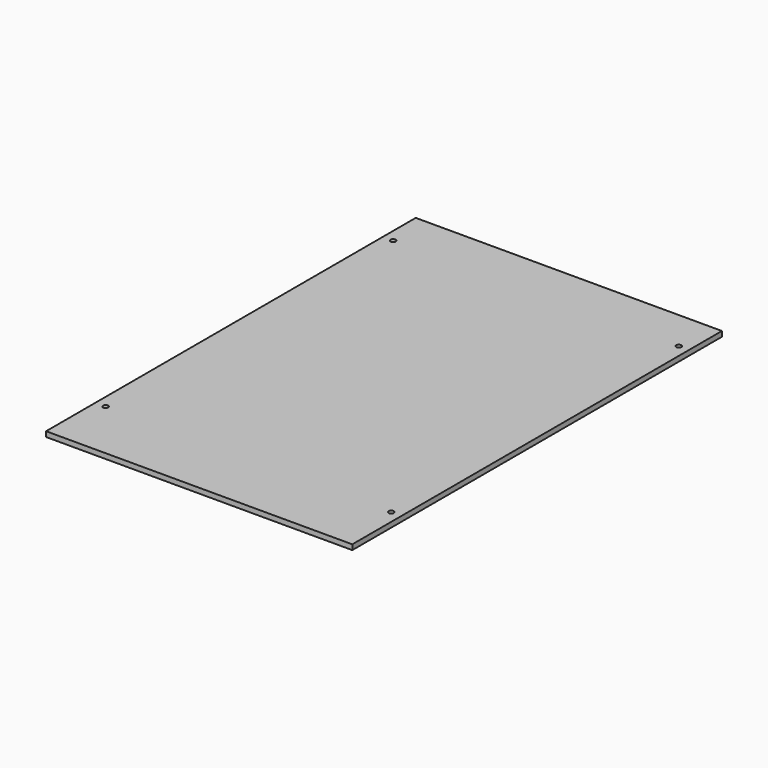
from build123d import *

# Parameters (mm, degrees)
F0_W     = 378.7394
F0_H     = 571.5
F1_DEPTH = 6.35
F3_DEPTH = 6.351


# Not quite as in the source:
# - a length typed as a fraction of an inch, garbled in the dataset ("3 / 203.2 mm" for 3/8 in), is restored


with BuildPart() as f1:
    # F0 (on Top) → F1 (new body)
    with BuildSketch(Plane.XY):
        with Locations((-22.0819663584, 200.0282000497)):
            Rectangle(F0_W, F0_H)
    extrude(amount=F1_DEPTH)

    # F2 (on face) → F3 (cut, through all)
    with BuildSketch(Plane.XY.offset(6.35)):
        with BuildLine():
            ThreePointArc((-201.9266663584, 434.9782000497), (-198.7516663584, 431.8032000497), (-195.5766663584, 434.9782000497))
            ThreePointArc((-195.5766663584, 434.9782000497), (-195.6025010735, 435.3824066906), (-195.679584789, 435.7800353388))
            Line((-195.679584789, 435.7800353388), (-198.7516663584, 434.9782000497))
            Line((-198.7516663584, 434.9782000497), (-201.9266663584, 434.9782000497))
        make_face()
        with BuildLine():
            Line((-198.7516663584, 434.9782000497), (-195.679584789, 435.7800353388))
            ThreePointArc((-195.679584789, 435.7800353388), (-196.8106874872, 437.4908134345), (-198.7516663584, 438.1532000497))
            Line((-198.7516663584, 438.1532000497), (-198.7516663584, 434.9782000497))
        make_face()
        with BuildLine():
            ThreePointArc((-198.7516663584, 438.1532000497), (-200.9967303887, 437.22326408), (-201.9266663584, 434.9782000497))
            Line((-201.9266663584, 434.9782000497), (-198.7516663584, 434.9782000497))
            Line((-198.7516663584, 434.9782000497), (-198.7516663584, 438.1532000497))
        make_face()
        with BuildLine():
            Line((154.5877336416, 434.9782000497), (157.7627336416, 434.9782000497))
            ThreePointArc((157.7627336416, 434.9782000497), (156.8327976718, 437.22326408), (154.5877336416, 438.1532000497))
            Line((154.5877336416, 438.1532000497), (154.5877336416, 434.9782000497))
        make_face()
        with BuildLine():
            ThreePointArc((154.5877336416, 438.1532000497), (152.3426696113, 432.7331360195), (157.7627336416, 434.9782000497))
            Line((157.7627336416, 434.9782000497), (154.5877336416, 434.9782000497))
            Line((154.5877336416, 434.9782000497), (154.5877336416, 438.1532000497))
        make_face()
        with BuildLine():
            ThreePointArc((-198.7516663584, -12.6967999503), (-196.5066023282, -11.7668639805), (-195.5766663584, -9.5217999503))
            ThreePointArc((-195.5766663584, -9.5217999503), (-196.5066023282, -7.27673592), (-198.7516663584, -6.3467999503))
            Line((-198.7516663584, -6.3467999503), (-198.7516663584, -9.5217999503))
            Line((-198.7516663584, -9.5217999503), (-198.7516663584, -12.6967999503))
        make_face()
        with BuildLine():
            Line((-198.7516663584, -9.5217999503), (-198.7516663584, -6.3467999503))
            ThreePointArc((-198.7516663584, -6.3467999503), (-200.9967303887, -7.27673592), (-201.9266663584, -9.5217999503))
            Line((-201.9266663584, -9.5217999503), (-198.7516663584, -9.5217999503))
        make_face()
        with BuildLine():
            ThreePointArc((-201.9266663584, -9.5217999503), (-200.9967303887, -11.7668639805), (-198.7516663584, -12.6967999503))
            Line((-198.7516663584, -12.6967999503), (-198.7516663584, -9.5217999503))
            Line((-198.7516663584, -9.5217999503), (-201.9266663584, -9.5217999503))
        make_face()
        with BuildLine():
            Line((154.5877336416, -9.5217999503), (157.7627336416, -9.5217999503))
            ThreePointArc((157.7627336416, -9.5217999503), (156.8327976718, -7.27673592), (154.5877336416, -6.3467999503))
            Line((154.5877336416, -6.3467999503), (154.5877336416, -9.5217999503))
        make_face()
        with BuildLine():
            ThreePointArc((154.5877336416, -12.6967999503), (156.8327976718, -11.7668639805), (157.7627336416, -9.5217999503))
            Line((157.7627336416, -9.5217999503), (154.5877336416, -9.5217999503))
            Line((154.5877336416, -9.5217999503), (154.5877336416, -12.6967999503))
        make_face()
        with BuildLine():
            Line((154.5877336416, -9.5217999503), (154.5877336416, -6.3467999503))
            ThreePointArc((154.5877336416, -6.3467999503), (151.4127336416, -9.5217999503), (154.5877336416, -12.6967999503))
            Line((154.5877336416, -12.6967999503), (154.5877336416, -9.5217999503))
        make_face()
    extrude(amount=-F3_DEPTH, mode=Mode.SUBTRACT)


solid = f1.part
